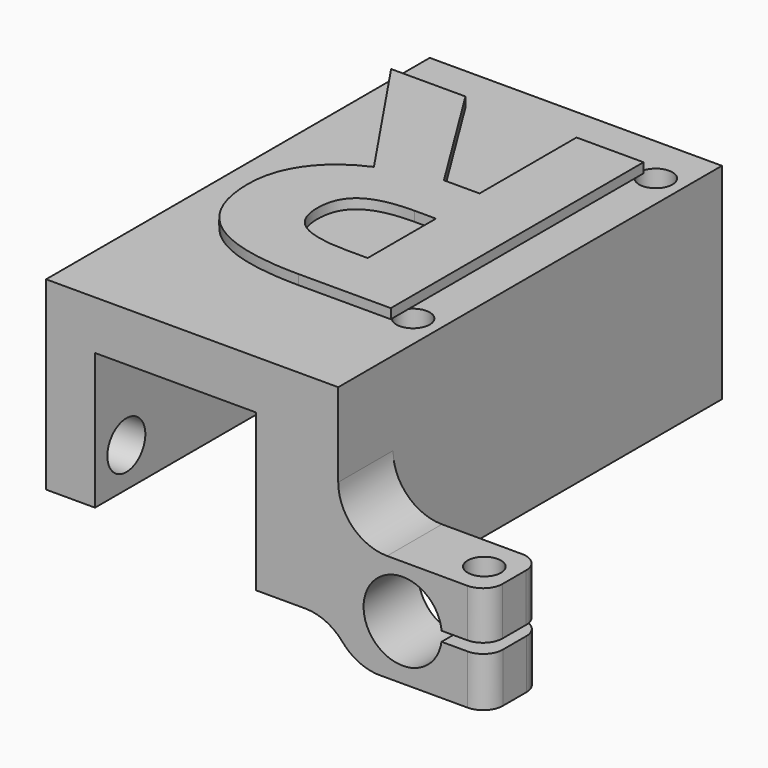
from build123d import *

# Parameters (mm, degrees)
F1_DEPTH      = 7
F2_DEPTH      = 42
F3_R          = 1.7
F3_R_2        = 11
F4_DEPTH      = 21.001
F5_R          = 4
F6_DEPTH      = 10
F7_DEPTH      = 21.001
F8_R          = 1.4
F9_DEPTH      = 11.0274245209
F8_R_2        = 1.7
F10_DEPTH     = 4.9110969969
F11_R         = 5
F12_R         = 5
F13_R         = 5
F14_R         = 2
F15_R         = 2.2
F15_R_2       = 2.4255023423
F16_DEPTH     = 6
F17_TEXT_SIZE = 45.2155919937
F18_DEPTH     = 1


# Not quite as in the source:
# - a feature names something its author has since deleted; it is built from what else it names
# - Text() gives the source's letters only with a copy of the font that has no kerning and outlines rounded to 1/6400 em; it was checked with that copy


with BuildPart() as f1:
    # F0 (on Front) → F1 (new body)
    with BuildSketch(Plane.XZ):
        Polygon((-24.9113007523, 29.8099789735), (-24.9113007523, 10.8925135386), (-19.9113007523, 10.8925135386), (-19.9113007523, 24.8099789735), (-3.4721007523, 24.8099789735), (-3.4721007523, 8.8099789735), (4.9380548998, 8.8099789735), (4.9380548998, 16.2656020473), (4.9380548998, 29.8099789735), align=None)
        Polygon((20.1263195603, 16.2417280634), (4.9380548998, 16.2656020473), (4.9380548998, 8.8099789735), (6.3533044869, 5.2860832236), (20.1553367778, 5.2860832236), (20.1553367778, 10.343908232), (13.4860510706, 10.343908232), (13.4860510706, 11.3388913612), (20.1263195603, 11.3388913612), align=None)
    extrude(amount=F1_DEPTH)

    # F0 (on Front) → F2 (join)
    with BuildSketch(Plane.XZ):
        Polygon((-24.9113007523, 29.8099789735), (-24.9113007523, 10.8925135386), (-19.9113007523, 10.8925135386), (-19.9113007523, 24.8099789735), (-3.4721007523, 24.8099789735), (-3.4721007523, 8.8099789735), (4.9380548998, 8.8099789735), (4.9380548998, 16.2656020473), (4.9380548998, 29.8099789735), align=None)
    extrude(amount=-F2_DEPTH)

    # F3 (on face) → F4 (cut, through all)
    with BuildSketch(Plane(origin=(0, 0, 8.8099789735), x_dir=(1, 0, 0), z_dir=(0, 0, -1))):
        with Locations((2.1850741468, -6)):
            Circle(F3_R)
        with Locations((2.1850741468, -37)):
            Circle(F3_R)
        with Locations((17.6850741468, -21.5)):
            Circle(F3_R_2)
    extrude(amount=-F4_DEPTH, mode=Mode.SUBTRACT)

    # F5 (on face) → F6 (cut)
    with BuildSketch(Plane.XZ.offset(7)):
        with Locations((11.5278992477, 10.8989789735)):
            Circle(F5_R)
    extrude(amount=-F6_DEPTH, mode=Mode.SUBTRACT)

    # F3 (on face) → F7 (cut, through all)
    with BuildSketch(Plane(origin=(0, 0, 8.8099789735), x_dir=(1, 0, 0), z_dir=(0, 0, -1))):
        with Locations((2.1850741468, -6)):
            Circle(F3_R)
        with Locations((2.1850741468, -37)):
            Circle(F3_R)
        with Locations((17.6850741468, -21.5)):
            Circle(F3_R_2)
    extrude(amount=-F7_DEPTH, mode=Mode.SUBTRACT)

    # F8 (on face) → F9 (cut, through all)
    with BuildSketch(Plane(origin=(0.0255795563, 0, 16.273323822), x_dir=(0.9999987646, 0, -0.0015718685), z_dir=(0.0015718685, 0, 0.9999987646))):
        with Locations((17.1007648362, -3.5767070949)):
            Circle(F8_R)
    extrude(amount=-F9_DEPTH, mode=Mode.SUBTRACT)

    # F8 (on face) → F10 (cut, through all)
    with BuildSketch(Plane(origin=(0.0255795563, 0, 16.273323822), x_dir=(0.9999987646, 0, -0.0015718685), z_dir=(0.0015718685, 0, 0.9999987646))):
        with Locations((17.1007648362, -3.5767070949)):
            Circle(F8_R_2)
        with Locations((17.1007648362, -3.5767070949)):
            Circle(F8_R, mode=Mode.SUBTRACT)
    extrude(amount=-F10_DEPTH, mode=Mode.SUBTRACT)

    # F11
    f11_edges = [f1.edges().sort_by_distance(p)[0] for p in [
        (4.938055, -3.5, 16.265602),
    ]]
    fillet(f11_edges, radius=F11_R)

    # F12
    f12_edges = [f1.edges().sort_by_distance(p)[0] for p in [
        (4.938055, -3.5, 8.809979),
    ]]
    fillet(f12_edges, radius=F12_R)

    # F13
    f13_edges = [f1.edges().sort_by_distance(p)[0] for p in [
        (6.353304, -3.5, 5.286083),
    ]]
    fillet(f13_edges, radius=F13_R)

    # F14
    f14_edges = [f1.edges().sort_by_distance(p)[0] for p in [
        (20.12632, -7, 13.79031),
        (20.155337, -7, 7.814996),
        (20.12632, 0, 13.79031),
        (20.155337, 0, 7.814996),
    ]]
    fillet(f14_edges, radius=F14_R)

    # F15 (on face) → F16 (cut)
    with BuildSketch(Plane(origin=(-24.9113007523, 0, 0), x_dir=(0, -1, 0), z_dir=(-1, 0, 0))):
        with Locations((-38, 14.8925135386)):
            Circle(F15_R)
        with Locations((3, 14.8925135386)):
            Circle(F15_R_2)
    extrude(amount=-F16_DEPTH, mode=Mode.SUBTRACT)

    # F17 (on face) → F18 (join)
    with BuildSketch(Plane.XY.offset(29.8099789735)):
        with Locations(Location((4.9380548998, 37.0661366887), (0, 0, 180))):
            Text('R', F17_TEXT_SIZE, font='Open Sans', font_style=FontStyle.BOLD, text_align=(TextAlign.LEFT, TextAlign.BOTTOM))
    extrude(amount=F18_DEPTH)


solid = f1.part
